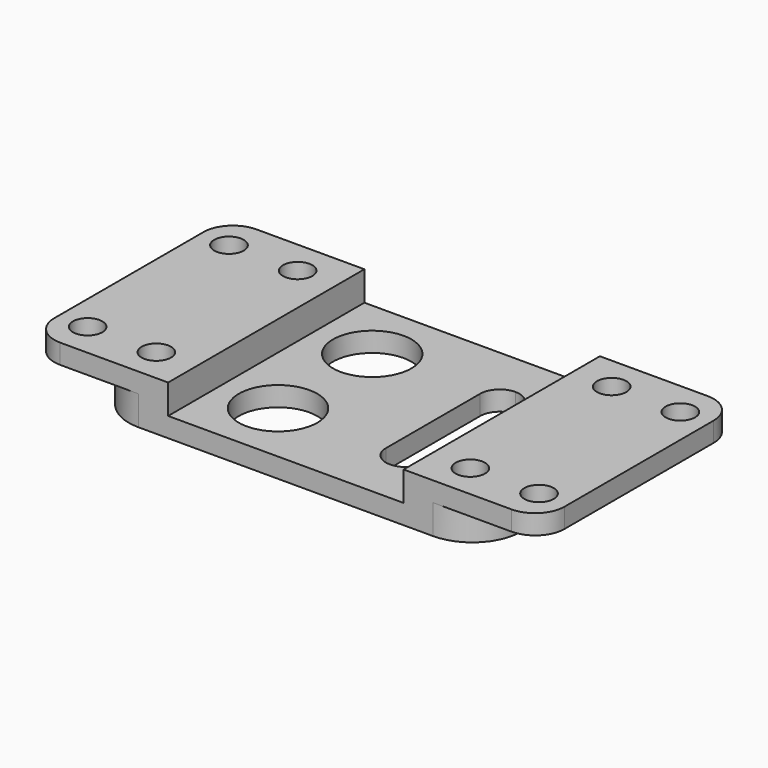
from build123d import *

# Parameters (mm, degrees)
F0_W      = 40
F0_H      = 25
F1_DEPTH  = 3
F2_R      = 5
F3_W      = 52
F3_H      = 25
F4_DEPTH  = 2
F5_R      = 3
F6_R      = 1.5
F7_DEPTH  = 25
F8_R      = 1.5
F9_DEPTH  = 4
F10_W     = 24
F10_H     = 25
F11_DEPTH = 3
F12_W     = 4
F12_H     = 16
F12_R     = 4
F13_DEPTH = 25
F14_R     = 1.99999


# Not quite as in the source:
# - a fillet or chamfer is up to 0.001 mm smaller than in the source, because OpenCascade refuses the exact size


with BuildPart() as f1:
    # F0 (on Top) → F1 (new body)
    with BuildSketch(Plane.XY):
        Rectangle(F0_W, F0_H)
    extrude(amount=F1_DEPTH)

    # F2
    f2_edges = [f1.edges().sort_by_distance(p)[0] for p in [
        (-20, -12.5, 1.5),
        (-20, 12.5, 1.5),
        (20, -12.5, 1.5),
        (20, 12.5, 1.5),
    ]]
    fillet(f2_edges, radius=F2_R)

    # F3 (on face) → F4 (join)
    with BuildSketch(Plane.XY.offset(3)):
        Rectangle(F3_W, F3_H)
    extrude(amount=F4_DEPTH)

    # F5
    f5_edges = [f1.edges().sort_by_distance(p)[0] for p in [
        (26, 12.5, 4),
        (26, -12.5, 4),
        (-26, -12.5, 4),
        (-26, 12.5, 4),
    ]]
    fillet(f5_edges, radius=F5_R)

    # F6 (on Top) → F7 (cut)
    with BuildSketch(Plane.XY):
        with Locations((23, 9)):
            Circle(F6_R)
        with Locations((23, -9)):
            Circle(F6_R)
        with Locations((-23, -9)):
            Circle(F6_R)
        with Locations((-23, 9)):
            Circle(F6_R)
    extrude(amount=F7_DEPTH, mode=Mode.SUBTRACT)

    # F8 (on face) → F9 (cut)
    with BuildSketch(Plane.XY.offset(5)):
        with Locations((16, -9)):
            Circle(F8_R)
        with Locations((-16, -9)):
            Circle(F8_R)
        with Locations((-16, 9)):
            Circle(F8_R)
        with Locations((16, 9)):
            Circle(F8_R)
    extrude(amount=-F9_DEPTH, mode=Mode.SUBTRACT)

    # F10 (on face) → F11 (cut)
    with BuildSketch(Plane.XY.offset(5)):
        Rectangle(F10_W, F10_H)
    extrude(amount=-F11_DEPTH, mode=Mode.SUBTRACT)

    # F12 (on face) → F13 (cut)
    with BuildSketch(Plane(origin=(0, 0, 0), x_dir=(1, 0, 0), z_dir=(0, 0, -1))):
        with Locations((7, 0)):
            Rectangle(F12_W, F12_H)
        with Locations((-6, -6)):
            Circle(F12_R)
        with Locations((-6, 6)):
            Circle(F12_R)
    extrude(amount=-F13_DEPTH, mode=Mode.SUBTRACT)

    # F14 (radius 2 in the source; OpenCascade refuses exactly that, so slightly less here)
    f14_edges = [f1.edges().sort_by_distance(p)[0] for p in [
        (9, 8, 1),
        (5, 8, 1),
        (9, -8, 1),
        (5, -8, 1),
    ]]
    fillet(f14_edges, radius=F14_R)


solid = f1.part
